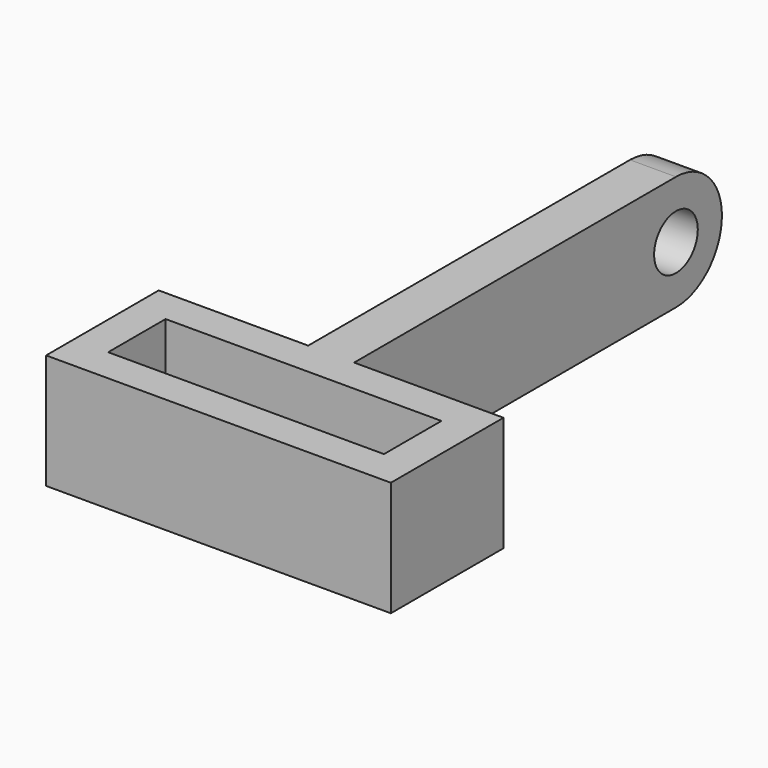
from build123d import *

# Parameters (mm, degrees)
F0_W     = 4
F0_H     = 40
F1_DEPTH = 10
F2_R     = 2.375
F3_DEPTH = 12.5
F4_R     = 4.99999


# Not quite as in the source:
# - a fillet or chamfer is up to 0.001 mm smaller than in the source, because OpenCascade refuses the exact size


with BuildPart() as f1:
    # F0 (on Top) → F1 (new body)
    with BuildSketch(Plane.XY):
        Polygon((-12.0077335707, 3), (-12.0077335707, 0), (11.9922664293, 0), (11.9922664293, -6.25), (14.9922664293, -6.25), (14.9922664293, 3), (2, 3), (-2, 3), align=None)
        Polygon((-12.0077335707, -6.25), (-12.0077335707, 0), (-12.0077335707, 3), (-15.0077335707, 3), (-15.0077335707, -9.25), (-12.0077335707, -9.25), align=None)
        Polygon((11.9922664293, -6.25), (-12.0077335707, -6.25), (-12.0077335707, -9.25), (14.9922664293, -9.25), (14.9922664293, -6.25), align=None)
        with Locations((0, 23)):
            Rectangle(F0_W, F0_H)
    extrude(amount=F1_DEPTH)

    # F2 (on Right) → F3 (cut, symmetric)
    with BuildSketch(Plane.YZ):
        with Locations((38, 5)):
            Circle(F2_R)
    extrude(amount=F3_DEPTH, both=True, mode=Mode.SUBTRACT)

    # F4 (radius 5 in the source; OpenCascade refuses exactly that, so slightly less here)
    f4_edges = [f1.edges().sort_by_distance(p)[0] for p in [
        (0, 43, 10),
        (0, 43, 0),
    ]]
    fillet(f4_edges, radius=F4_R)


solid = f1.part
